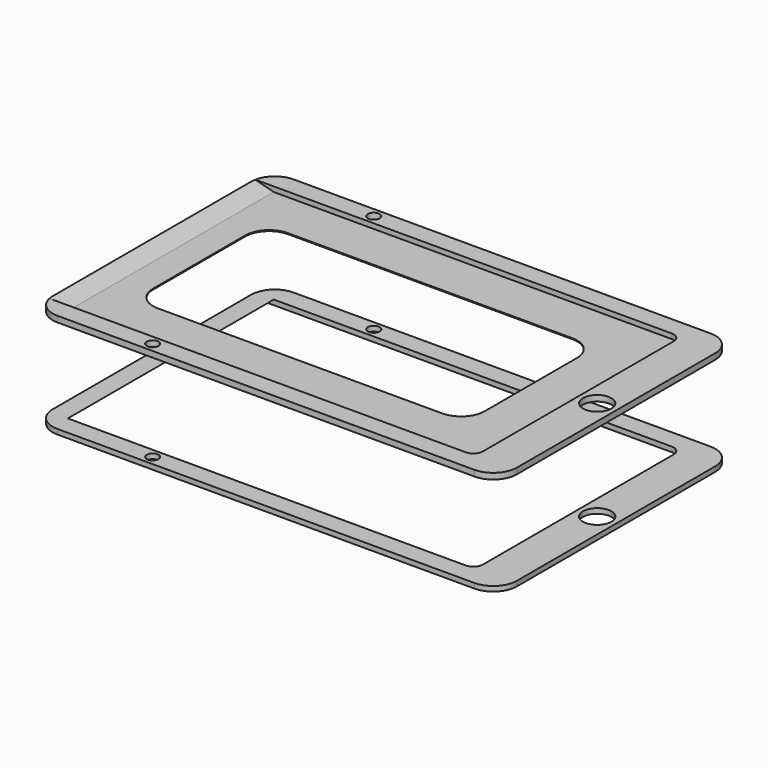
from build123d import *

# Parameters (mm, degrees)
F1_R        = 1.25
F1_R_2      = 3
F2_DEPTH    = 1.05
F5_T1_DEPTH = 26.05
F8_R        = 1.25
F8_R_2      = 3
F9_DEPTH    = 0.2


# Not quite as in the source:
# - a fillet or chamfer that OpenCascade refuses, or shapes differently, is made with other operations: its cross-section is extruded or revolved along the edge and cut away or added


with BuildPart() as f2:
    # F1 (on Top) → F2 (new body)
    with BuildSketch(Plane.XY):
        with BuildLine():
            Line((-47.05, 27.2), (-43.05, 27.2))
            Line((-43.05, 27.2), (41.05, 27.2))
            ThreePointArc((41.05, 27.2), (42.4642135624, 26.6142135624), (43.05, 25.2))
            Line((43.05, 25.2), (43.05, -25.2))
            ThreePointArc((43.05, -25.2), (42.4642135624, -26.6142135624), (41.05, -27.2))
            Line((41.05, -27.2), (-43.05, -27.2))
            Line((-43.05, -27.2), (-47.05, -27.2))
            Line((-47.05, -27.2), (-47.05, -31.2))
            Line((-47.05, -31.2), (51.05, -31.2))
            Line((51.05, -31.2), (51.05, 31.2))
            Line((51.05, 31.2), (-47.05, 31.2))
            Line((-47.05, 31.2), (-47.05, 27.2))
        make_face()
        with Locations((-23.525, -29.2)):
            Circle(F1_R, mode=Mode.SUBTRACT)
        with Locations((-23.525, 29.2)):
            Circle(F1_R, mode=Mode.SUBTRACT)
        with Locations((47.05, 0)):
            Circle(F1_R_2, mode=Mode.SUBTRACT)
    extrude(amount=F2_DEPTH)

    # F4: sweep along a path in F1
    with BuildLine(Plane.XY) as f4_path:
        Line((-47.05, -27.2), (-47.05, 27.2))
    # F3 (on face) → F4 (sweep)
    with BuildSketch(Plane(origin=(0, -27.2, 0), x_dir=(-1, 0, 0), z_dir=(0, 1, 0))):
        Polygon((47.05, 1.05), (43.05, 0), (47.05, 0), align=None)
    sweep(path=f4_path.line)

    # F5: fillet of radius 5 on 4 edges, made by hand

    # F5_s2 → F5_t1 (cut)
    with BuildSketch(Plane.XY.offset(-12.5)):
        with BuildLine():
            ThreePointArc((-42.05, 31.2), (-45.5855339059, 29.7355339059), (-47.05, 26.2))
            Line((-47.05, 26.2), (-47.05, 31.2))
            Line((-47.05, 31.2), (-42.05, 31.2))
        make_face()
        with BuildLine():
            ThreePointArc((-42.05, -31.2), (-45.5855339059, -29.7355339059), (-47.05, -26.2))
            Line((-47.05, -26.2), (-47.05, -31.2))
            Line((-47.05, -31.2), (-42.05, -31.2))
        make_face()
        with BuildLine():
            ThreePointArc((46.05, 31.2), (49.5855339059, 29.7355339059), (51.05, 26.2))
            Line((51.05, 26.2), (51.05, 31.2))
            Line((51.05, 31.2), (46.05, 31.2))
        make_face()
        with BuildLine():
            ThreePointArc((51.05, -26.2), (49.5855339059, -29.7355339059), (46.05, -31.2))
            Line((46.05, -31.2), (51.05, -31.2))
            Line((51.05, -31.2), (51.05, -26.2))
        make_face()
    extrude(amount=F5_T1_DEPTH, mode=Mode.SUBTRACT)


with BuildPart() as f7_1:
    # F7: instance of F2
    add(f2.part.mirror(Plane.XY.offset(-10)))


with BuildPart() as f2_1:
    add(f2.part)

    # F8 (on face) → F9 (join)
    with BuildSketch(Plane.XY):
        with BuildLine():
            Line((-42.05, -31.2), (46.05, -31.2))
            ThreePointArc((46.05, -31.2), (49.5855339059, -29.7355339059), (51.05, -26.2))
            Line((51.05, -26.2), (51.05, 26.2))
            ThreePointArc((51.05, 26.2), (49.5855339059, 29.7355339059), (46.05, 31.2))
            Line((46.05, 31.2), (-42.05, 31.2))
            ThreePointArc((-42.05, 31.2), (-45.5855339059, 29.7355339059), (-47.05, 26.2))
            Line((-47.05, 26.2), (-47.05, -26.2))
            ThreePointArc((-47.05, -26.2), (-45.5855339059, -29.7355339059), (-42.05, -31.2))
        make_face()
        with Locations((-23.525, -29.2)):
            Circle(F8_R, mode=Mode.SUBTRACT)
        with BuildLine():
            ThreePointArc((33.05, -12.2), (31.5855339059, -15.7355339059), (28.05, -17.2))
            Line((28.05, -17.2), (-32.05, -17.2))
            ThreePointArc((-32.05, -17.2), (-35.5855339059, -15.7355339059), (-37.05, -12.2))
            Line((-37.05, -12.2), (-37.05, 12.2))
            ThreePointArc((-37.05, 12.2), (-35.5855339059, 15.7355339059), (-32.05, 17.2))
            Line((-32.05, 17.2), (28.05, 17.2))
            ThreePointArc((28.05, 17.2), (31.5855339059, 15.7355339059), (33.05, 12.2))
            Line((33.05, 12.2), (33.05, -12.2))
        make_face(mode=Mode.SUBTRACT)
        with Locations((-23.525, 29.2)):
            Circle(F8_R, mode=Mode.SUBTRACT)
        with Locations((47.05, 0)):
            Circle(F8_R_2, mode=Mode.SUBTRACT)
    extrude(amount=-F9_DEPTH)


solid = Compound([f7_1.part, f2_1.part])
